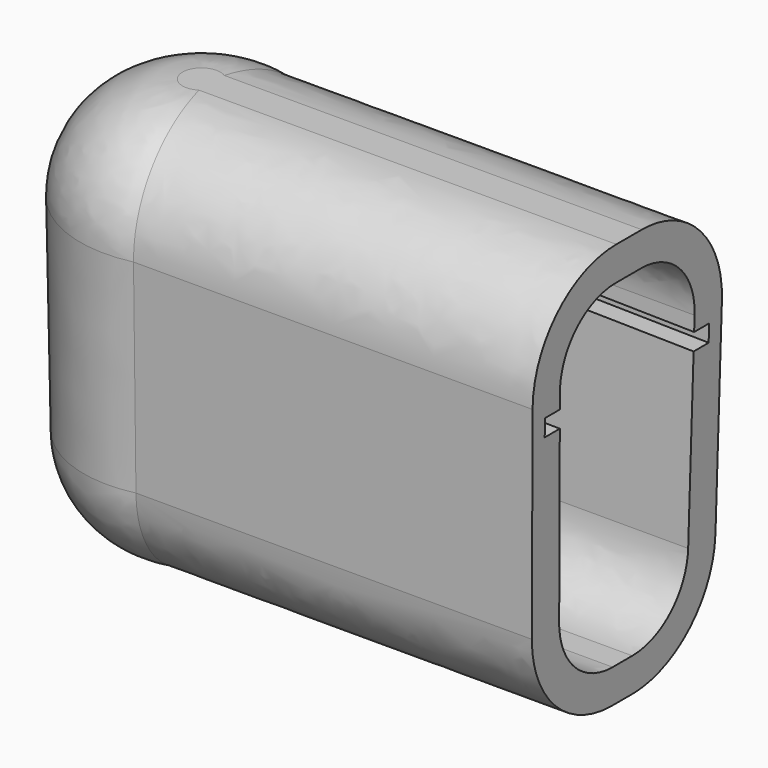
from build123d import *

# Parameters (mm, degrees)
F0_R          = 100
F1_DEPTH      = 200
F1_TAPER      = -1
F1_DEPTH_BACK = 200
F1_TAPER_BACK = 1
F2_W          = 500
F2_H          = 200
F3_DEPTH      = 400
F3_TAPER      = 1
F4_R          = 80
F5_T          = 40
F6_W          = 240
F6_H          = 20
F7_DEPTH      = 500


with BuildPart() as f1:
    # F0 (on Top) → F1 (new body, two sides)
    with BuildSketch(Plane.XY) as f1_sk:
        Circle(F0_R)
    extrude(amount=F1_DEPTH, taper=F1_TAPER)
    extrude(f1_sk.sketch, amount=-F1_DEPTH_BACK, taper=F1_TAPER_BACK)

    # F2 (on face) → F3 (join, through all)
    with BuildSketch(Plane.XY.offset(200)):
        with Locations((250, 0)):
            Rectangle(F2_W, F2_H)
    extrude(amount=-F3_DEPTH, taper=F3_TAPER)

    # F4
    f4_edges = [f1.edges().sort_by_distance(p)[0] for p in [
        (263.326569, -100, 200),
        (263.326569, 100, 200),
        (259.370179, -93.017974, -200),
        (259.370179, 93.017974, -200),
        (-96.508987, 0, -200),
        (-103.491013, 0, 200),
    ]]
    fillet(f4_edges, radius=F4_R)

    # F5
    f5_openings = [f1.faces().sort_by_distance(p)[0] for p in [
        (496.54488, 0, 2.056321),
    ]]
    offset(amount=F5_T, openings=f5_openings)

    # F6 (on face) → F7 (cut)
    with BuildSketch(Plane(origin=(496.3577570845, 0, -8.6639568775), x_dir=(0, 1, 0), z_dir=(0.9998476952, 0, -0.0174524064))):
        with Locations((0, 100)):
            Rectangle(F6_W, F6_H)
    extrude(amount=-F7_DEPTH, mode=Mode.SUBTRACT)


solid = f1.part
